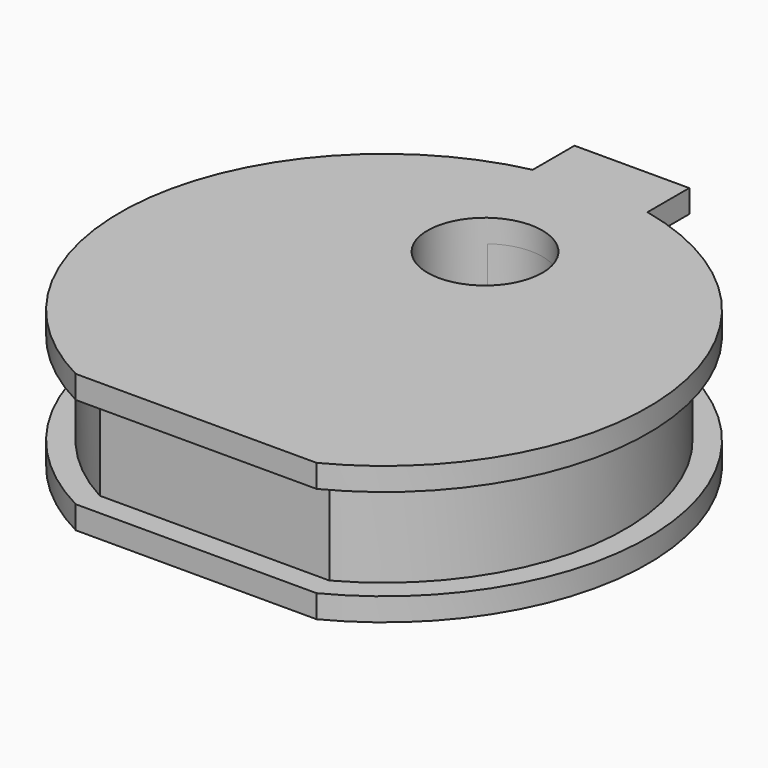
from build123d import *

# Parameters (mm, degrees)
F1_DEPTH      = 4
F4_DEPTH      = 1
F5_DEPTH      = 1
F6_R          = 2.5
F7_DEPTH      = 1.001
F7_DEPTH_BACK = 5.001


with BuildPart() as f1:
    # F0 (on Top) → F1 (new body)
    with BuildSketch(Plane.XY):
        with BuildLine():
            Line((-5, -9.233093), (5, -9.233093))
            ThreePointArc((5, -9.233093), (10.336903, 1.843487), (1.5, 10.392305))
            Line((1.5, 10.392305), (1.5, 7.5))
            ThreePointArc((1.5, 7.5), (2.236068, 6.618034), (2.5, 5.5))
            ThreePointArc((2.5, 5.5), (-1.118034, 3.263932), (-1.5, 7.5))
            Line((-1.5, 7.5), (-1.5, 10.392305))
            ThreePointArc((-1.5, 10.392305), (-10.336903, 1.843487), (-5, -9.233093))
        make_face()
        with BuildLine():
            Line((1.5, 7.5), (1.5, 10.392305))
            ThreePointArc((1.5, 10.392305), (0, 10.5), (-1.5, 10.392305))
            Line((-1.5, 10.392305), (-1.5, 7.5))
            ThreePointArc((-1.5, 7.5), (0, 8), (1.5, 7.5))
        make_face()
        with BuildLine():
            ThreePointArc((-1.5, 10.392305), (0, 10.5), (1.5, 10.392305))
            Line((1.5, 10.392305), (1.5, 12.5))
            Line((1.5, 12.5), (-1.5, 12.5))
            Line((-1.5, 12.5), (-1.5, 10.392305))
        make_face()
    extrude(amount=F1_DEPTH)

    # F2 (on face) → F4 (join)
    with BuildSketch(Plane.XY.offset(4)):
        with BuildLine():
            Line((2.5, 13.5), (-2.5, 13.5))
            Line((-2.5, 13.5), (-2.5, 11.224972))
            ThreePointArc((-2.5, 11.224972), (-11.406892, 1.46042), (-5.247267, -10.233093))
            Line((-5.247267, -10.233093), (5.247267, -10.233093))
            ThreePointArc((5.247267, -10.233093), (11.406892, 1.46042), (2.5, 11.224972))
            Line((2.5, 11.224972), (2.5, 13.5))
        make_face()
    extrude(amount=F4_DEPTH)

    # F3 (on face) → F5 (join)
    with BuildSketch(Plane(origin=(0, 0, 0), x_dir=(1, 0, 0), z_dir=(0, 0, -1))):
        with BuildLine():
            Line((5.247267, 10.233093), (-5.247267, 10.233093))
            ThreePointArc((-5.247267, 10.233093), (-11.406892, -1.46042), (-2.5, -11.224972))
            Line((-2.5, -11.224972), (-2.5, -13.5))
            Line((-2.5, -13.5), (2.5, -13.5))
            Line((2.5, -13.5), (2.5, -11.224972))
            ThreePointArc((2.5, -11.224972), (11.406892, -1.46042), (5.247267, 10.233093))
        make_face()
    extrude(amount=F5_DEPTH)

    # F6 (on Top) → F7 (cut, two sides)
    with BuildSketch(Plane.XY) as f7_sk:
        with Locations((0, 5.5)):
            Circle(F6_R)
    extrude(amount=-F7_DEPTH, mode=Mode.SUBTRACT)
    extrude(f7_sk.sketch, amount=F7_DEPTH_BACK, mode=Mode.SUBTRACT)


solid = f1.part
